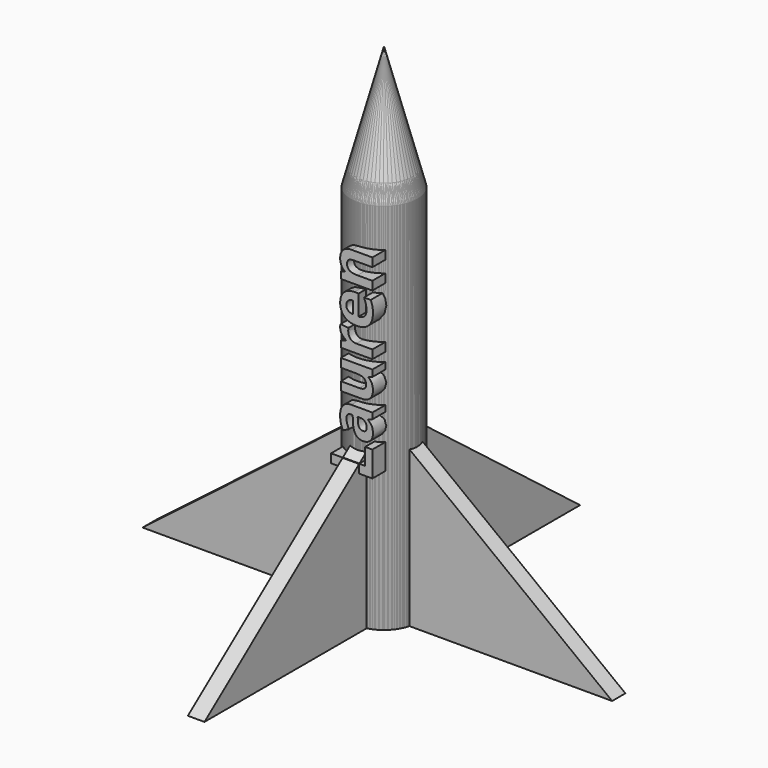
from build123d import *

# Parameters (mm, degrees)
F0_R         = 25.4
F1_DEPTH     = 381
F2_SIZE2     = 94.7940905122
F2_SIZE      = 25.4
F4_DEPTH     = 6.35
F5_COUNT     = 4
F6_TEXT_SIZE = 44.3758753439
F7_DEPTH     = 31.75


# Not quite as in the source:
# - Text() gives the source's letters only with a copy of the font that has no kerning and outlines rounded to 1/6400 em; it was checked with that copy


with BuildPart() as f1:
    # F0 (on Top) → F1 (new body)
    with BuildSketch(Plane.XY):
        Circle(F0_R)
    extrude(amount=F1_DEPTH)

    # F2
    f2_edges = [f1.edges().sort_by_distance(p)[0] for p in [
        (-25.4, 0, 381),
    ]]
    f2_side = f1.faces().sort_by_distance((0, 0, 381))[0]
    chamfer(f2_edges, length=F2_SIZE, length2=F2_SIZE2, reference=f2_side)

    # F3 (on Front) → F4 (join, symmetric)
    with BuildSketch(Plane.XZ):
        Polygon((180.0248473883, 0), (0, 138.2333636284), (0, 0), align=None)
    extrude(amount=F4_DEPTH, both=True)


with BuildPart() as f5_1:
    # F5: instance of F1
    add(f1.part.rotate(Axis((0, 0, 0), (0, 0, -1)), 1 * 360 / F5_COUNT))


with BuildPart() as f5_2:
    # F5: instance of F1
    add(f1.part.rotate(Axis((0, 0, 0), (0, 0, -1)), 2 * 360 / F5_COUNT))


with BuildPart() as f5_3:
    # F5: instance of F1
    add(f1.part.rotate(Axis((0, 0, 0), (0, 0, -1)), 3 * 360 / F5_COUNT))


with BuildPart() as f7:
    # F6 (on Front) → F7 (new body)
    with BuildSketch(Plane.XZ):
        with Locations(Location((16.474539414, 103.3402998), (0, 0, 90))):
            Text('Lauren', F6_TEXT_SIZE, font='Open Sans', font_style=FontStyle.BOLD, text_align=(TextAlign.LEFT, TextAlign.BOTTOM))
    extrude(amount=F7_DEPTH)


solid = Compound([f1.part, f5_1.part, f5_2.part, f5_3.part, f7.part])
